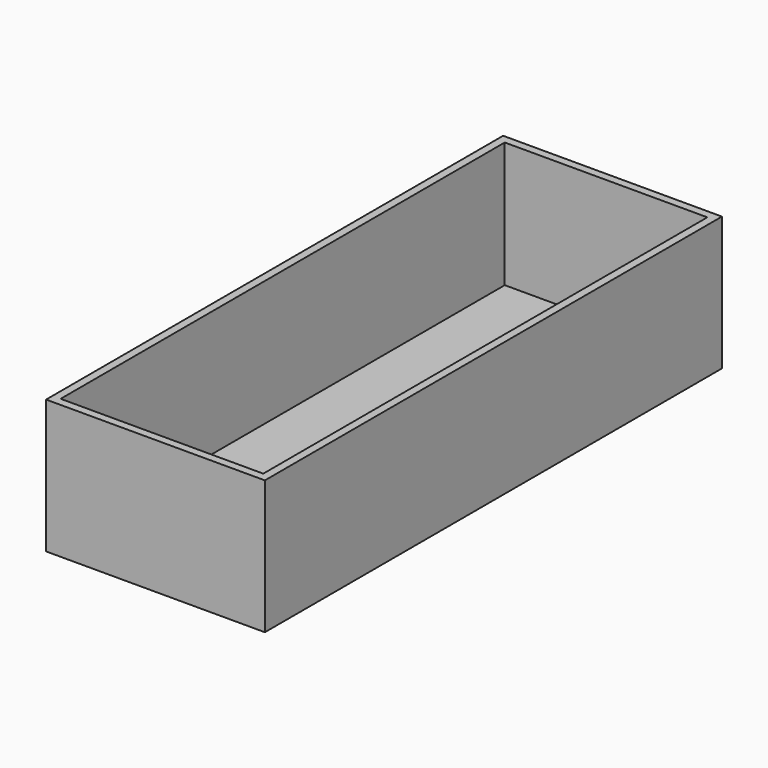
from build123d import *

# Parameters (mm, degrees)
F0_W     = 54
F0_H     = 141
F0_W_2   = 50
F0_H_2   = 137
F1_DEPTH = 33
F2_W     = 54
F2_H     = 2
F3_DEPTH = 141


# Not quite as in the source:
# - the program builds the solid bodies; features that only make, move or delete a surface that nothing else refers to are left out


with BuildPart() as f1:
    # F0 (on Top) → F1 (new body)
    with BuildSketch(Plane.XY):
        with Locations((27, 70.5)):
            Rectangle(F0_W, F0_H)
        with Locations((27, 70.5)):
            Rectangle(F0_W_2, F0_H_2, mode=Mode.SUBTRACT)
    extrude(amount=F1_DEPTH)

    # F2 (on face) → F3 (join)
    with BuildSketch(Plane.XZ):
        with Locations((27, 1)):
            Rectangle(F2_W, F2_H)
    extrude(amount=-F3_DEPTH)


solid = f1.part
